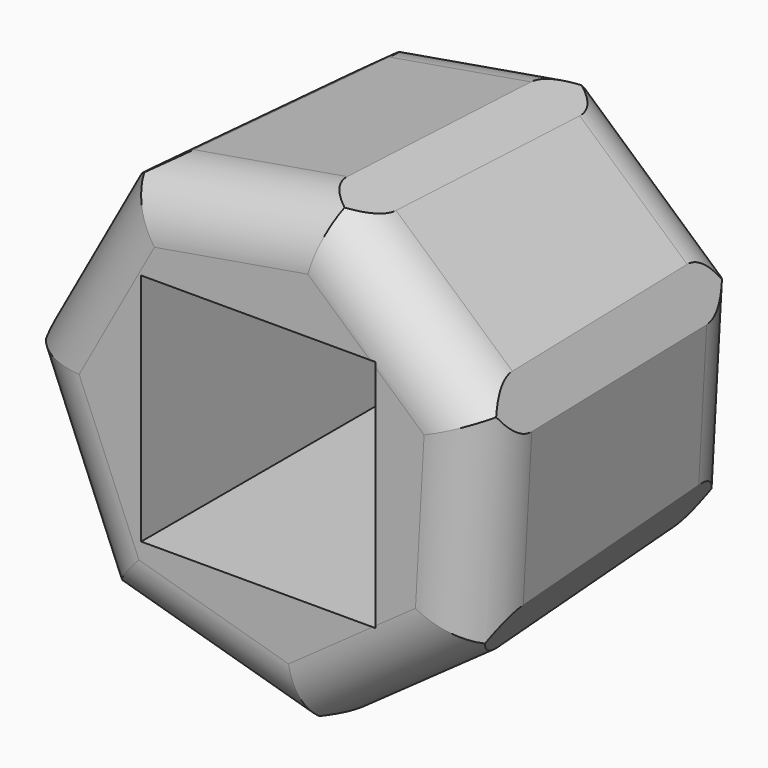
from build123d import *

# Parameters (mm, degrees)
F1_DEPTH               = 30
DRAFT_F1_DRAFTED_ANGLE = -3
F2_R                   = 5
F3_R                   = 5
F4_W                   = 20
F4_H                   = 20
F5_DEPTH               = 25
F6_T1_DEPTH            = 32.9613742489
F6_T3_DEPTH            = 32.9613742489
F6_T5_DEPTH            = 32.9613742489
F6_T7_DEPTH            = 32.9613742489
F6_T9_DEPTH            = 32.9613742489
F6_T11_DEPTH           = 32.9613742489
F6_T13_DEPTH           = 32.9613742489


# Not quite as in the source:
# - a fillet or chamfer that OpenCascade refuses, or shapes differently, is made with other operations: its cross-section is extruded or revolved along the edge and cut away or added
# - an extrude with a draft is written as a straight extrude whose walls are then drafted


with BuildPart() as f1:
    # F0 (on Front) → F1 (new body)
    with BuildSketch(Plane.XZ):
        Polygon((17.9385137087, 7.4487195661), (5.3608368971, 18.6690954525), (-11.2536594392, 15.8312616831), (-19.393920685, 1.0721649674), (-12.9301640911, -14.4942938369), (3.2702697907, -19.1462537523), (17.0081238187, -9.3806940798), align=None)
    extrude(amount=F1_DEPTH)

    # draft_F1_drafted
    draft_f1_drafted_walls = [f1.faces().sort_by_distance(p)[0] for p in [
        (11.6496753029, -20, 13.0589075093),
        (-2.9464112711, -20, 17.2501785678),
        (-15.3237900621, -20, 8.4517133252),
        (-16.162042388, -20, -6.7110644348),
        (-4.8299471502, -20, -16.8202737946),
        (10.1391968047, -20, -14.2634739161),
        (17.4733187637, -20, -0.9659872569),
    ]]
    draft(draft_f1_drafted_walls, neutral_plane=Plane.XZ, angle=DRAFT_F1_DRAFTED_ANGLE)

    # F2
    f2_edges = [f1.edges().sort_by_distance(p)[0] for p in [
        (12.696304, -30, 14.232145),
        (-3.211122, -30, 18.799968),
        (-16.700509, -30, 9.211031),
        (-17.614071, -30, -7.313999),
        (-5.263879, -30, -18.331439),
        (11.050122, -30, -15.544932),
        (19.043155, -30, -1.052773),
    ]]
    fillet(f2_edges, radius=F2_R)

    # F3
    f3_edges = [f1.edges().sort_by_distance(p)[0] for p in [
        (11.649675, 0, 13.058908),
        (-2.946411, 0, 17.250179),
        (-15.32379, 0, 8.451713),
        (-16.162042, 0, -6.711064),
        (-4.829947, 0, -16.820274),
        (10.139197, 0, -14.263474),
        (17.473319, 0, -0.965987),
    ]]
    fillet(f3_edges, radius=F3_R)

    # F4 (on face) → F5 (cut)
    with BuildSketch(Plane.XZ.offset(30)):
        Rectangle(F4_W, F4_H)
    extrude(amount=-F5_DEPTH, mode=Mode.SUBTRACT)

    # F6: chamfer of 5 on 7 edges, made by hand

    # F6_s2 → F6_t1 (cut)
    with BuildSketch(Plane(origin=(-0.0316165808, 0.5885328858, -0.0131283476), x_dir=(0.9985601423, 0.0536436589, 0), z_dir=(0.0536303558, -0.9983125086, 0.0222692631))):
        with BuildLine():
            Line((16.0443324574, 9.2126584741), (17.8567326718, 4.8405349345))
            Line((17.8567326718, 4.8405349345), (17.95658055, 4.8350212048))
            ThreePointArc((17.95658055, 4.8350212048), (17.9412936163, 6.1298642359), (18.0125326805, 7.4199291889))
            Line((18.0125326805, 7.4199291889), (17.979348174, 7.4999814647))
            ThreePointArc((17.979348174, 7.4999814647), (17.0162874881, 8.3612925017), (16.1109958291, 9.2871970203))
            Line((16.1109958291, 9.2871970203), (16.0443324574, 9.2126584741))
        make_face()
    extrude(amount=F6_T1_DEPTH, mode=Mode.SUBTRACT)

    # F6_s4 → F6_t3 (cut)
    with BuildSketch(Plane(origin=(-0.0094484602, 0.5885328858, -0.0329042291), x_dir=(0.9998711553, 0.0160521919, 0), z_dir=(0.016027169, -0.9983125086, 0.055814559))):
        with BuildLine():
            Line((7.3464704277, 16.980078104), (2.7979979647, 18.2883812174))
            Line((2.7979979647, 18.2883812174), (2.7812705799, 18.3869722646))
            ThreePointArc((2.7812705799, 18.3869722646), (4.0695924821, 18.5176583078), (5.3434187967, 18.7337812066))
            Line((5.3434187967, 18.7337812066), (5.4266999686, 18.7098265674))
            ThreePointArc((5.4266999686, 18.7098265674), (6.3910250601, 17.8499313964), (7.4130242149, 17.0547145121))
            Line((7.4130242149, 17.0547145121), (7.3464704277, 16.980078104))
        make_face()
    extrude(amount=F6_T3_DEPTH, mode=Mode.SUBTRACT)

    # F6_s6 → F6_t5 (cut)
    with BuildSketch(Plane(origin=(-0.0299767712, 0.5885328858, 0.0165334474), x_dir=(0.9987053445, 0.0508687999, 0), z_dir=(0.0508487909, -0.9983125086, -0.0280452422))):
        with BuildLine():
            Line((17.2151289641, -6.7773899779), (14.9323145776, -10.9233539501))
            Line((14.9323145776, -10.9233539501), (14.9903647621, -11.0047798433))
            ThreePointArc((14.9903647621, -11.0047798433), (15.9921070393, -10.1841918983), (17.0441543428, -9.4341658599))
            Line((17.0441543428, -9.4341658599), (17.0859519922, -9.3582544981))
            ThreePointArc((17.0859519922, -9.3582544981), (17.1572014154, -8.0681901173), (17.3149767981, -6.7829045093))
            Line((17.3149767981, -6.7829045093), (17.2151289641, -6.7773899779))
        make_face()
    extrude(amount=F6_T5_DEPTH, mode=Mode.SUBTRACT)

    # F6_s8 → F6_t7 (cut)
    with BuildSketch(Plane(origin=(0.0198345436, 0.5885328858, -0.0279025549), x_dir=(0.9994325819, -0.0336825513, 0), z_dir=(-0.033644803, -0.9983125086, 0.0473303536))):
        with BuildLine():
            Line((-8.7154535169, 16.3197595006), (-12.5708343582, 13.5745277525))
            Line((-12.5708343582, 13.5745277525), (-12.6584055319, 13.6228111816))
            ThreePointArc((-12.6584055319, 13.6228111816), (-11.9586816709, 14.7124160107), (-11.3348450828, 15.8438622085))
            Line((-11.3348450828, 15.8438622085), (-11.2642542114, 15.8941265817))
            ThreePointArc((-11.2642542114, 15.8941265817), (-9.9909866351, 16.1135172521), (-8.7324338192, 16.4183073029))
            Line((-8.7324338192, 16.4183073029), (-8.7154535169, 16.3197595006))
        make_face()
    extrude(amount=F6_T7_DEPTH, mode=Mode.SUBTRACT)

    # F6_s10 → F6_t9 (cut)
    with BuildSketch(Plane(origin=(-0.0057638415, 0.5885328858, 0.0337452193), x_dir=(0.9999520464, 0.0097931062, 0), z_dir=(0.0097770493, -0.9983125086, -0.057241108))):
        with BuildLine():
            Line((5.4270153992, -17.6873170385), (0.7619123903, -18.4854853783))
            Line((0.7619123903, -18.4854853783), (0.7344030916, -18.5816271408))
            ThreePointArc((0.7344030916, -18.5816271408), (2.0004228609, -18.853741288), (3.2426036707, -19.2091697938))
            Line((3.2426036707, -19.2091697938), (3.3280203132, -19.1945555699))
            ThreePointArc((3.3280203132, -19.1945555699), (4.3813809063, -18.4463750783), (5.4849227429, -17.7688445771))
            Line((5.4849227429, -17.7688445771), (5.4270153992, -17.6873170385))
        make_face()
    extrude(amount=F6_T9_DEPTH, mode=Mode.SUBTRACT)

    # F6_s12 → F6_t11 (cut)
    with BuildSketch(Plane(origin=(0.0341817315, 0.5885328858, -0.0018896878), x_dir=(0.9983176374, -0.05798185, 0), z_dir=(-0.0579815521, -0.9983125086, 0.0032054266))):
        with BuildLine():
            Line((-18.1909247679, 3.3740089286), (-18.451737393, -1.3516905495))
            Line((-18.451737393, -1.3516905495), (-18.544113645, -1.38998713))
            ThreePointArc((-18.544113645, -1.38998713), (-18.9588658626, -0.1632708778), (-19.4536693294, 1.0302583913))
            Line((-19.4536693294, 1.0302583913), (-19.4488939282, 1.116784537))
            ThreePointArc((-19.4488939282, 1.116784537), (-18.8257532782, 2.2486141697), (-18.2785256186, 3.4222384937))
            Line((-18.2785256186, 3.4222384937), (-18.1909247679, 3.3740089286))
        make_face()
    extrude(amount=F6_T11_DEPTH, mode=Mode.SUBTRACT)

    # F6_s14 → F6_t13 (cut)
    with BuildSketch(Plane(origin=(0.0227893784, 0.5885328858, 0.0255461528), x_dir=(0.9992511317, -0.0386933555, 0), z_dir=(-0.0386570098, -0.9983125086, -0.043333252))):
        with BuildLine():
            Line((-10.4619030107, -15.2591698843), (-13.9910517613, -12.1055421513))
            Line((-13.9910517613, -12.1055421513), (-14.0834131593, -12.1438745416))
            ThreePointArc((-14.0834131593, -12.1438745416), (-13.5081086408, -13.3039938787), (-13.0128424993, -14.497331231))
            Line((-13.0128424993, -14.497331231), (-12.94822484, -14.5550732126))
            ThreePointArc((-12.94822484, -14.5550732126), (-11.7069147347, -14.9135307547), (-10.4896467494, -15.3552442563))
            Line((-10.4896467494, -15.3552442563), (-10.4619030107, -15.2591698843))
        make_face()
    extrude(amount=F6_T13_DEPTH, mode=Mode.SUBTRACT)


solid = f1.part
